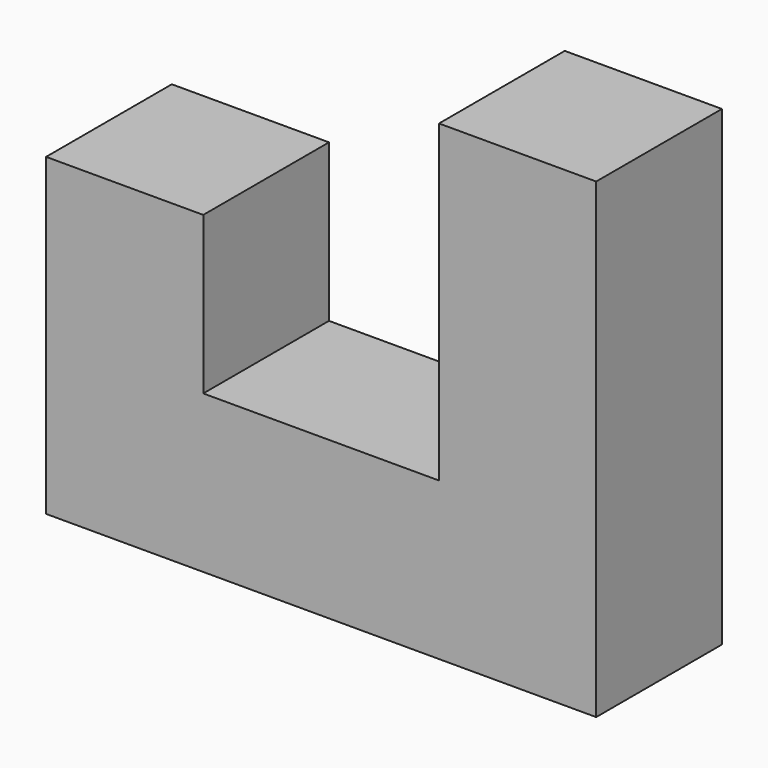
from build123d import *

# Parameters (mm, degrees)
F1_DEPTH = 25.4


# Not quite as in the source:
# - ends of sketch curves that miss each other by under 0.0002 mm in the source are joined


with BuildPart() as f1:
    # F0 (on Front) → F1 (new body)
    with BuildSketch(Plane.XZ):
        Polygon((-60.5589975275, 13.4836168304), (-60.5589975275, -37.3163831696), (28.3410024725, -37.3163831696), (28.3410024725, 38.8836168304), (2.9410024725, 38.883614792), (2.9410065494, -11.916385208), (-35.1589975275, -11.9163831696), (-35.1589975275, 13.4836168304), align=None)
    extrude(amount=F1_DEPTH)


solid = f1.part
